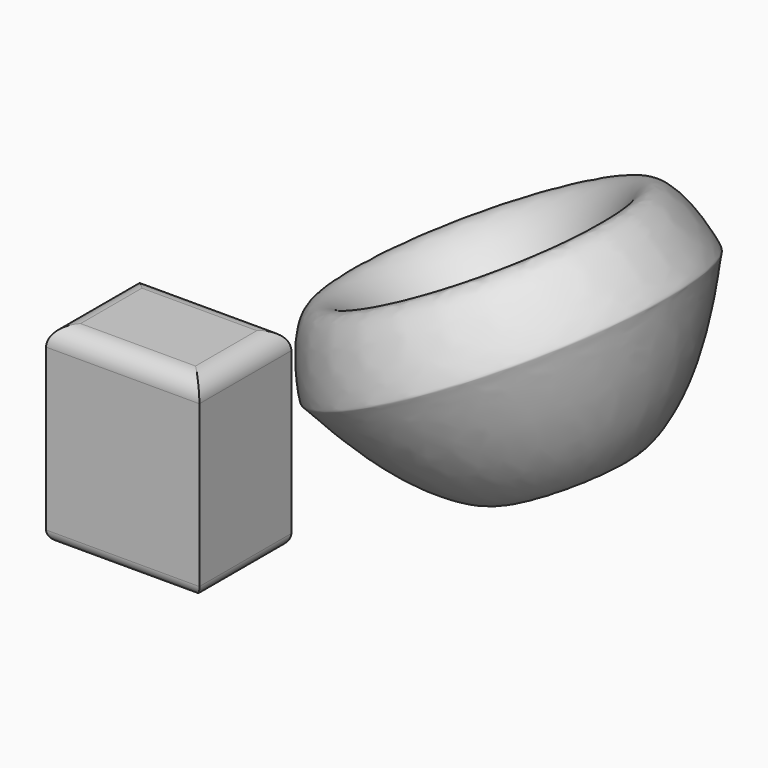
from build123d import *

# Parameters (mm, degrees)
F0_W     = 101.6
F0_H     = 127
F2_DEPTH = 76.2
F3_R     = 12.7
F4_R     = 7.62


# Not quite as in the source:
# - a feature names something its author has since deleted; it is built from what else it names


with BuildPart() as f1:
    # F0 (on Front) → F1 (revolve)
    with BuildSketch(Plane.XZ):
        with BuildLine():
            add(Edge.make_bspline(
                [(0, 67.6398426294), (13.3935718053, 74.3762328832), (42.8956839394, 37.7354229944), (41.1346471608, 36.1149227712), (41.7408109301, -31.509032611), (-14.011665596, -117.9732392774), (-22.2011812589, 56.4736038375), (0, 67.6398426294)],
                knots=[0, 0, 0, 0, 0.1966106986, 0.2485014456, 0.4799841226, 0.6740981553, 1, 1, 1, 1], degree=3))
        make_face()
    revolve(axis=Axis((-91.6760973632, 0, 45.9895678796), (0.4393510153, 0, -0.898315471)))


with BuildPart() as f2:
    # F0 (on Front) → F2 (new body)
    with BuildSketch(Plane.XZ):
        with Locations((-258.9270345211, -126.4065781832)):
            Rectangle(F0_W, F0_H)
    extrude(amount=F2_DEPTH)

    # F3
    f3_edges = [f2.edges().sort_by_distance(p)[0] for p in [
        (-258.927035, 0, -62.906578),
        (-309.727035, -38.1, -62.906578),
        (-258.927035, -76.2, -62.906578),
        (-208.127035, -38.1, -62.906578),
    ]]
    fillet(f3_edges, radius=F3_R)

    # F4
    f4_edges = [f2.edges().sort_by_distance(p)[0] for p in [
        (-258.927035, -76.2, -189.906578),
        (-309.727035, -38.1, -189.906578),
        (-258.927035, 0, -189.906578),
        (-208.127035, -38.1, -189.906578),
    ]]
    fillet(f4_edges, radius=F4_R)


solid = Compound([f1.part, f2.part])
